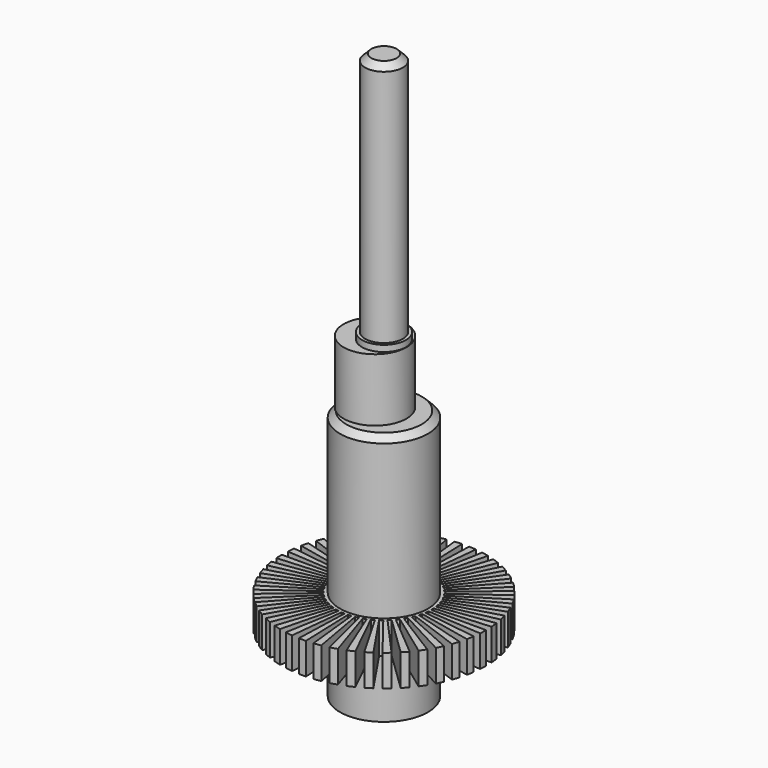
from build123d import *

# Parameters (mm, degrees)
F0_R             = 1.5
F1_DEPTH         = 25
F2_R             = 2.5
F3_DEPTH         = 5
F4_R             = 1.75
F5_DEPTH         = 0.5
F6_R             = 3.5
F7_DEPTH         = 20
F8_W             = 8.125
F8_H             = 2.5
F10_R            = 2.5
F11_DEPTH        = 13
F12_S9_R         = 2.5
F12_T10_DEPTH    = 6
F14_DEPTH        = 7.251
F14_COPIES_COUNT = 45


# Not quite as in the source:
# - a fillet or chamfer that OpenCascade refuses, or shapes differently, is made with other operations: its cross-section is extruded or revolved along the edge and cut away or added
# - a pattern or mirror of a feature is missing from the dataset's text; its kind, count and spacing are read off the source's solid


with BuildPart() as f1:
    # F0 (on Top) → F1 (new body)
    with BuildSketch(Plane.XY):
        Circle(F0_R)
    extrude(amount=F1_DEPTH)

    # F2 (on face) → F3 (join)
    with BuildSketch(Plane(origin=(0, 0, 0), x_dir=(1, 0, 0), z_dir=(0, 0, -1))):
        with Locations((-0.714, 0)):
            Circle(F2_R)
    extrude(amount=-F3_DEPTH)

    # F4 (on face) → F5 (join)
    with BuildSketch(Plane.XY.offset(5)):
        Circle(F4_R)
    extrude(amount=F5_DEPTH)

    # F6 (on face) → F7 (join)
    with BuildSketch(Plane(origin=(0, 0, 0), x_dir=(1, 0, 0), z_dir=(0, 0, -1))):
        Circle(F6_R)
    extrude(amount=F7_DEPTH)

    # F8 (on Front) → F9 (revolve)
    with BuildSketch(Plane.XZ):
        with Locations((4.0625, -14)):
            Rectangle(F8_W, F8_H)
    revolve(axis=Axis((0, 0, -10.8621492982), (0, 0, -1)))

    # F10 (on face) → F11 (cut)
    with BuildSketch(Plane(origin=(0, 0, -20), x_dir=(1, 0, 0), z_dir=(0, 0, -1))):
        Circle(F10_R)
    extrude(amount=-F11_DEPTH, mode=Mode.SUBTRACT)

    # F12: chamfer of 0.5 on 3 edges, made by hand

    # F12_s1 → F12_t2 (revolve, cut)
    with BuildSketch(Plane.XZ):
        Polygon((1.5, 24.5), (1, 25), (1.5, 25), align=None)
    revolve(axis=Axis((0, 0, 25), (0, 0, 1)), mode=Mode.SUBTRACT)

    # F12_s3 → F12_t4 (revolve, cut)
    with BuildSketch(Plane.XZ):
        Polygon((3, -20), (2.5, -19.5), (2.5, -20), align=None)
    revolve(axis=Axis((0, 0, -20), (0, 0, -1)), mode=Mode.SUBTRACT)


with BuildPart() as f12_tool6:
    # F12_s7 → F12_t8 (revolve)
    with BuildSketch(Plane.XZ):
        Polygon((3.5, -0.5), (3, 0), (3.5, 0), align=None)
    revolve(axis=Axis((0, 0, 0), (0, 0, -1)))

    # F12_s9 → F12_t10 (cut, symmetric)
    with BuildSketch(Plane.XY.offset(-0.2)):
        with Locations((-0.714, 0)):
            Circle(F12_S9_R)
    extrude(amount=F12_T10_DEPTH, both=True, mode=Mode.SUBTRACT)


with BuildPart() as f1_1:
    add(f1.part)

    # F12_t5: cut F12_tool6
    add(f12_tool6.part, mode=Mode.SUBTRACT)

    # F13 (on face) → F14 (cut, through all)
    with BuildSketch(Plane.XY.offset(-12.75)):
        with BuildLine():
            Line((-0.2835584107, 8.1200504695), (-0.1308731126, 3.7477156013))
            ThreePointArc((-0.1308731126, 3.7477156013), (0, 3.75), (0.1308731126, 3.7477156013))
            Line((0.1308731126, 3.7477156013), (0.2835584107, 8.1200504695))
            ThreePointArc((0.2835584107, 8.1200504695), (0, 8.125), (-0.2835584107, 8.1200504695))
        make_face()
    f14 = extrude(amount=-F14_DEPTH, mode=Mode.SUBTRACT)

    # F14_copies: F14 ×45 about axis
    f14_copies_axis = Axis((0, 0, 0), (0, 0, 1))
    for i in range(1, F14_COPIES_COUNT):
        add(f14.rotate(f14_copies_axis, i * 360 / F14_COPIES_COUNT), mode=Mode.SUBTRACT)


solid = f1_1.part
